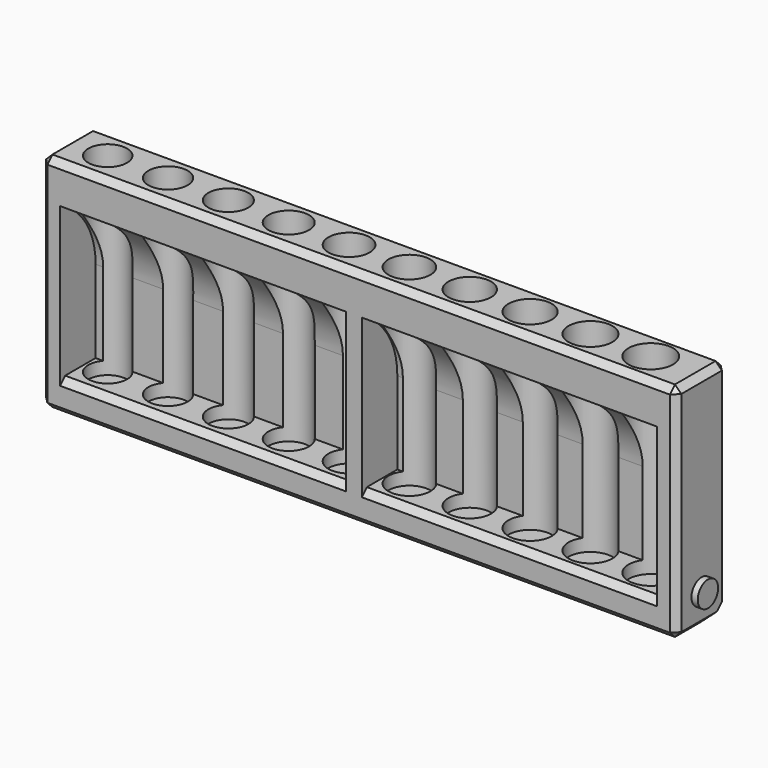
from build123d import *

# Parameters (mm, degrees)
F0_W          = 100
F0_H          = 10
F2_DEPTH      = 35
F3_START      = 3
F1_R          = 3.5
F1_R_2        = 3.45
F1_R_3        = 3.4
F1_R_4        = 3.35
F1_R_5        = 3.3
F1_R_6        = 3.25
F1_R_7        = 3.2
F1_R_8        = 3.15
F1_R_9        = 3.1
F1_R_10       = 3.05
F3_DEPTH      = 37
F5_START      = -3
F5_DEPTH      = 46.5
F6_START      = -52
F6_DEPTH      = 45
F7_SIZE       = 1
F8_R          = 2
F9_DEPTH      = 2
F9_DEPTH_BACK = 1
F10_START     = -99
F10_DEPTH     = 2
F11_T1_DEPTH  = 123


# Not quite as in the source:
# - a fillet or chamfer that OpenCascade refuses, or shapes differently, is made with other operations: its cross-section is extruded or revolved along the edge and cut away or added


with BuildPart() as f2:
    # F0 (on Top) → F2 (new body)
    with BuildSketch(Plane.XY):
        with Locations((-50, -5)):
            Rectangle(F0_W, F0_H)
    extrude(amount=F2_DEPTH)

    # F1 (on Top) → F3 (cut)
    with BuildSketch(Plane.XY.offset(F3_START)):
        with Locations((-8, -5)):
            Circle(F1_R)
        with Locations((-17.5, -5)):
            Circle(F1_R_2)
        with Locations((-27, -5)):
            Circle(F1_R_3)
        with Locations((-36.5, -5)):
            Circle(F1_R_4)
        with Locations((-46, -5)):
            Circle(F1_R_5)
        with Locations((-55.5, -5)):
            Circle(F1_R_6)
        with Locations((-65, -5)):
            Circle(F1_R_7)
        with Locations((-74.5, -5)):
            Circle(F1_R_8)
        with Locations((-84, -5)):
            Circle(F1_R_9)
        with Locations((-93.5, -5)):
            Circle(F1_R_10)
    extrude(amount=F3_DEPTH, mode=Mode.SUBTRACT)

    # F4 (on Right) → F5 (cut)
    with BuildSketch(Plane.YZ.offset(F5_START)):
        with BuildLine():
            Line((-13, 29.8321595662), (-13, 5))
            Line((-13, 5), (-3, 5))
            Line((-3, 5), (-3, 18))
            ThreePointArc((-3, 18), (-5.8348486101, 25.7459666924), (-13, 29.8321595662))
        make_face()
        with BuildLine():
            ThreePointArc((-15, 30), (-13.9964848766, 29.9579662735), (-13, 29.8321595662))
            Line((-13, 29.8321595662), (-13, 30))
            Line((-13, 30), (-15, 30))
        make_face()
    extrude(amount=-F5_DEPTH, mode=Mode.SUBTRACT)

    # F4 (on Right) → F6 (cut)
    with BuildSketch(Plane.YZ.offset(F6_START)):
        with BuildLine():
            Line((-13, 29.8321595662), (-13, 5))
            Line((-13, 5), (-3, 5))
            Line((-3, 5), (-3, 18))
            ThreePointArc((-3, 18), (-5.8348486101, 25.7459666924), (-13, 29.8321595662))
        make_face()
        with BuildLine():
            ThreePointArc((-15, 30), (-13.9964848766, 29.9579662735), (-13, 29.8321595662))
            Line((-13, 29.8321595662), (-13, 30))
            Line((-13, 30), (-15, 30))
        make_face()
    extrude(amount=-F6_DEPTH, mode=Mode.SUBTRACT)

    # F7
    f7_edges = [f2.edges().sort_by_distance(p)[0] for p in [
        (-50, -10, 35),
        (-100, -5, 35),
        (-50, 0, 35),
        (0, -5, 35),
        (0, -10, 17.5),
        (0, 0, 17.5),
        (0, -5, 0),
        (-50, -10, 0),
        (-100, -10, 17.5),
        (-74.5, -10, 5),
        (-26.25, -10, 5),
        (-100, -5, 0),
        (-100, 0, 17.5),
    ]]
    chamfer(f7_edges, length=F7_SIZE)

    # F8 (on Right) → F9 (join, two sides)
    with BuildSketch(Plane.YZ) as f9_sk:
        with Locations((-5, 5)):
            Circle(F8_R)
    extrude(amount=-F9_DEPTH)
    extrude(f9_sk.sketch, amount=F9_DEPTH_BACK)

    # F8 (on Right) → F10 (join)
    with BuildSketch(Plane.YZ.offset(F10_START)):
        with Locations((-5, 5)):
            Circle(F8_R)
    extrude(amount=-F10_DEPTH)

    # F11: fillet of radius 5 on 1 edges, made by hand

    # F11_s2 → F11_t1 (cut)
    with BuildSketch(Plane.YZ.offset(-111.5)):
        with BuildLine():
            ThreePointArc((0, 5), (-1.4644660941, 1.4644660941), (-5, 0))
            Line((-5, 0), (0, 0))
            Line((0, 0), (0, 5))
        make_face()
    extrude(amount=F11_T1_DEPTH, mode=Mode.SUBTRACT)


solid = f2.part
